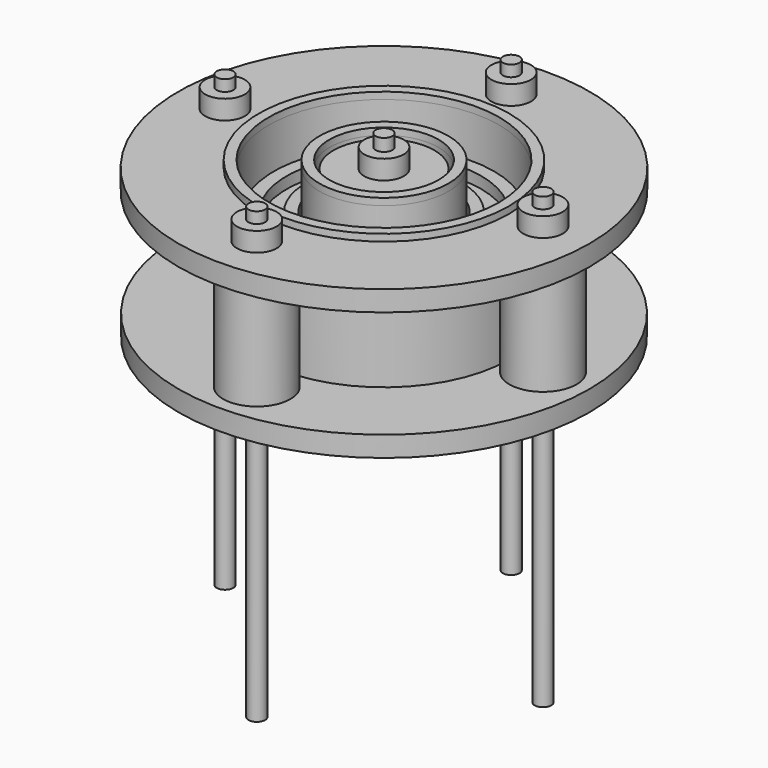
from build123d import *

# Parameters (mm, degrees)
F0_R           = 64.3
F0_R_2         = 10.5
F0_R_3         = 39.15
F0_R_4         = 6.2
F0_R_5         = 2.6
F1_DEPTH       = 6.4
F0_R_6         = 36.015
F2_DEPTH       = 46.5
F2_DEPTH_BACK  = 2.15
F3_R           = 64.2044551284
F3_R_2         = 39.15
F3_R_3         = 36.015
F4_DEPTH       = 6.4
F0_R_7         = 20.15
F0_R_8         = 17.07
F5_DEPTH       = 40.1
F5_DEPTH_BACK  = 2.15
F0_R_9         = 34.415
F0_R_10        = 30.415
F0_R_11        = 24.415
F0_R_12        = 20.915
F6_DEPTH       = 40.1
F7_DEPTH       = 12.2
F8_DEPTH       = 15.8
F9_DEPTH       = 12.2
F10_START      = -0.35
F0_R_13        = 15.75
F10_DEPTH      = 39.75
F11_DEPTH      = 6
F12_DEPTH      = 131
F12_DEPTH_BACK = 9.5
F13_START      = -6.4
F13_DEPTH      = 33.7
F14_DEPTH      = 65.9
F14_DEPTH_BACK = 9.5
F15_DEPTH      = 5.65
F15_DEPTH_BACK = 0.35


with BuildPart() as f1:
    # F0 (on Top) → F1 (new body)
    with BuildSketch(Plane.XY):
        Circle(F0_R)
        with Locations((0, -49.7)):
            Circle(F0_R_2, mode=Mode.SUBTRACT)
        with Locations((-49.7, 0)):
            Circle(F0_R_2, mode=Mode.SUBTRACT)
        Circle(F0_R_3, mode=Mode.SUBTRACT)
        with Locations((49.7, 0)):
            Circle(F0_R_2, mode=Mode.SUBTRACT)
        with Locations((0, 49.7)):
            Circle(F0_R_2, mode=Mode.SUBTRACT)
        with Locations((0, -49.7)):
            Circle(F0_R_2)
        with Locations((0, -49.7)):
            Circle(F0_R_4, mode=Mode.SUBTRACT)
        with Locations((49.7, 0)):
            Circle(F0_R_2)
        with Locations((49.7, 0)):
            Circle(F0_R_4, mode=Mode.SUBTRACT)
        with Locations((0, 49.7)):
            Circle(F0_R_2)
        with Locations((0, 49.7)):
            Circle(F0_R_4, mode=Mode.SUBTRACT)
        with Locations((-49.7, 0)):
            Circle(F0_R_2)
        with Locations((-49.7, 0)):
            Circle(F0_R_4, mode=Mode.SUBTRACT)
        with Locations((0, -49.7)):
            Circle(F0_R_4)
        with Locations((0, -49.7)):
            Circle(F0_R_5, mode=Mode.SUBTRACT)
        with Locations((49.7, 0)):
            Circle(F0_R_4)
        with Locations((49.7, 0)):
            Circle(F0_R_5, mode=Mode.SUBTRACT)
        with Locations((0, 49.7)):
            Circle(F0_R_4)
        with Locations((0, 49.7)):
            Circle(F0_R_5, mode=Mode.SUBTRACT)
        with Locations((-49.7, 0)):
            Circle(F0_R_4)
        with Locations((-49.7, 0)):
            Circle(F0_R_5, mode=Mode.SUBTRACT)
    extrude(amount=-F1_DEPTH)

    # F0 (on Top) → F11 (join)
    with BuildSketch(Plane.XY):
        with Locations((49.7, 0)):
            Circle(F0_R_4)
        with Locations((49.7, 0)):
            Circle(F0_R_5, mode=Mode.SUBTRACT)
        with Locations((0, -49.7)):
            Circle(F0_R_4)
        with Locations((0, -49.7)):
            Circle(F0_R_5, mode=Mode.SUBTRACT)
        with Locations((-49.7, 0)):
            Circle(F0_R_4)
        with Locations((-49.7, 0)):
            Circle(F0_R_5, mode=Mode.SUBTRACT)
        with Locations((0, 49.7)):
            Circle(F0_R_4)
        with Locations((0, 49.7)):
            Circle(F0_R_5, mode=Mode.SUBTRACT)
    extrude(amount=F11_DEPTH)


with BuildPart() as f2:
    # F0 (on Top) → F2 (new body, two sides)
    with BuildSketch(Plane.XY) as f2_sk:
        Circle(F0_R_3)
        Circle(F0_R_6, mode=Mode.SUBTRACT)
    extrude(amount=-F2_DEPTH)
    extrude(f2_sk.sketch, amount=F2_DEPTH_BACK)

    # F3 (on face) → F4 (join)
    with BuildSketch(Plane(origin=(0, 0, -46.5), x_dir=(1, 0, 0), z_dir=(0, 0, -1))):
        Circle(F3_R)
        Circle(F3_R_2, mode=Mode.SUBTRACT)
        Circle(F3_R_2)
        Circle(F3_R_3, mode=Mode.SUBTRACT)
        Circle(F3_R_3)
    extrude(amount=-F4_DEPTH)


with BuildPart() as f5:
    # F0 (on Top) → F5 (new body, two sides)
    with BuildSketch(Plane.XY) as f5_sk:
        Circle(F0_R_7)
        Circle(F0_R_8, mode=Mode.SUBTRACT)
    extrude(amount=-F5_DEPTH)
    extrude(f5_sk.sketch, amount=F5_DEPTH_BACK)


with BuildPart() as f6:
    # F0 (on Top) → F6 (new body)
    with BuildSketch(Plane.XY):
        Circle(F0_R_9)
        Circle(F0_R_10, mode=Mode.SUBTRACT)
        Circle(F0_R_10)
        Circle(F0_R_11, mode=Mode.SUBTRACT)
        Circle(F0_R_11)
        Circle(F0_R_12, mode=Mode.SUBTRACT)
    extrude(amount=-F6_DEPTH)

    # F0 (on Top) → F7 (cut)
    with BuildSketch(Plane.XY):
        Circle(F0_R_9)
        Circle(F0_R_10, mode=Mode.SUBTRACT)
    extrude(amount=-F7_DEPTH, mode=Mode.SUBTRACT)

    # F0 (on Top) → F8 (cut)
    with BuildSketch(Plane.XY):
        Circle(F0_R_10)
        Circle(F0_R_11, mode=Mode.SUBTRACT)
    extrude(amount=-F8_DEPTH, mode=Mode.SUBTRACT)

    # F0 (on Top) → F9 (cut)
    with BuildSketch(Plane.XY):
        Circle(F0_R_11)
        Circle(F0_R_12, mode=Mode.SUBTRACT)
    extrude(amount=-F9_DEPTH, mode=Mode.SUBTRACT)


with BuildPart() as f10:
    # F0 (on Top) → F10 (new body)
    with BuildSketch(Plane.XY.offset(F10_START)):
        Circle(F0_R_13)
        Circle(F0_R_4, mode=Mode.SUBTRACT)
        Circle(F0_R_4)
        Circle(F0_R_5, mode=Mode.SUBTRACT)
    extrude(amount=-F10_DEPTH)


with BuildPart() as f12:
    # F0 (on Top) → F12 (new body, two sides)
    with BuildSketch(Plane.XY) as f12_sk:
        with Locations((-49.7, 0)):
            Circle(F0_R_5)
    extrude(amount=-F12_DEPTH)
    extrude(f12_sk.sketch, amount=F12_DEPTH_BACK)


with BuildPart() as f12b:
    # F0 (on Top) → F12, piece 2 (new body, two sides)
    with BuildSketch(Plane.XY) as f12_2_sk:
        with Locations((0, 49.7)):
            Circle(F0_R_5)
    extrude(amount=-F12_DEPTH)
    extrude(f12_2_sk.sketch, amount=F12_DEPTH_BACK)


with BuildPart() as f12c:
    # F0 (on Top) → F12, piece 3 (new body, two sides)
    with BuildSketch(Plane.XY) as f12_3_sk:
        with Locations((49.7, 0)):
            Circle(F0_R_5)
    extrude(amount=-F12_DEPTH)
    extrude(f12_3_sk.sketch, amount=F12_DEPTH_BACK)


with BuildPart() as f12d:
    # F0 (on Top) → F12, piece 4 (new body, two sides)
    with BuildSketch(Plane.XY) as f12_4_sk:
        with Locations((0, -49.7)):
            Circle(F0_R_5)
    extrude(amount=-F12_DEPTH)
    extrude(f12_4_sk.sketch, amount=F12_DEPTH_BACK)


with BuildPart() as f13:
    # F0 (on Top) → F13 (new body)
    with BuildSketch(Plane.XY.offset(F13_START)):
        with Locations((0, -49.7)):
            Circle(F0_R_2)
        with Locations((0, -49.7)):
            Circle(F0_R_4, mode=Mode.SUBTRACT)
        with Locations((0, -49.7)):
            Circle(F0_R_4)
        with Locations((0, -49.7)):
            Circle(F0_R_5, mode=Mode.SUBTRACT)
    extrude(amount=-F13_DEPTH)


with BuildPart() as f13b:
    # F0 (on Top) → F13, piece 2 (new body)
    with BuildSketch(Plane.XY.offset(F13_START)):
        with Locations((0, 49.7)):
            Circle(F0_R_2)
        with Locations((0, 49.7)):
            Circle(F0_R_4, mode=Mode.SUBTRACT)
        with Locations((0, 49.7)):
            Circle(F0_R_4)
        with Locations((0, 49.7)):
            Circle(F0_R_5, mode=Mode.SUBTRACT)
    extrude(amount=-F13_DEPTH)


with BuildPart() as f13c:
    # F0 (on Top) → F13, piece 3 (new body)
    with BuildSketch(Plane.XY.offset(F13_START)):
        with Locations((-49.7, 0)):
            Circle(F0_R_2)
        with Locations((-49.7, 0)):
            Circle(F0_R_4, mode=Mode.SUBTRACT)
        with Locations((-49.7, 0)):
            Circle(F0_R_4)
        with Locations((-49.7, 0)):
            Circle(F0_R_5, mode=Mode.SUBTRACT)
    extrude(amount=-F13_DEPTH)


with BuildPart() as f13d:
    # F0 (on Top) → F13, piece 4 (new body)
    with BuildSketch(Plane.XY.offset(F13_START)):
        with Locations((49.7, 0)):
            Circle(F0_R_2)
        with Locations((49.7, 0)):
            Circle(F0_R_4, mode=Mode.SUBTRACT)
        with Locations((49.7, 0)):
            Circle(F0_R_4)
        with Locations((49.7, 0)):
            Circle(F0_R_5, mode=Mode.SUBTRACT)
    extrude(amount=-F13_DEPTH)


with BuildPart() as f14:
    # F0 (on Top) → F14 (new body, two sides)
    with BuildSketch(Plane.XY) as f14_sk:
        Circle(F0_R_5)
    extrude(amount=-F14_DEPTH)
    extrude(f14_sk.sketch, amount=F14_DEPTH_BACK)


with BuildPart() as f15:
    # F0 (on Top) → F15 (new body, two sides)
    with BuildSketch(Plane.XY) as f15_sk:
        Circle(F0_R_4)
        Circle(F0_R_5, mode=Mode.SUBTRACT)
    extrude(amount=F15_DEPTH)
    extrude(f15_sk.sketch, amount=-F15_DEPTH_BACK)


solid = Compound([f1.part, f2.part, f5.part, f6.part, f10.part, f12.part, f12b.part, f12c.part, f12d.part, f13.part, f13b.part, f13c.part, f13d.part, f14.part, f15.part])
